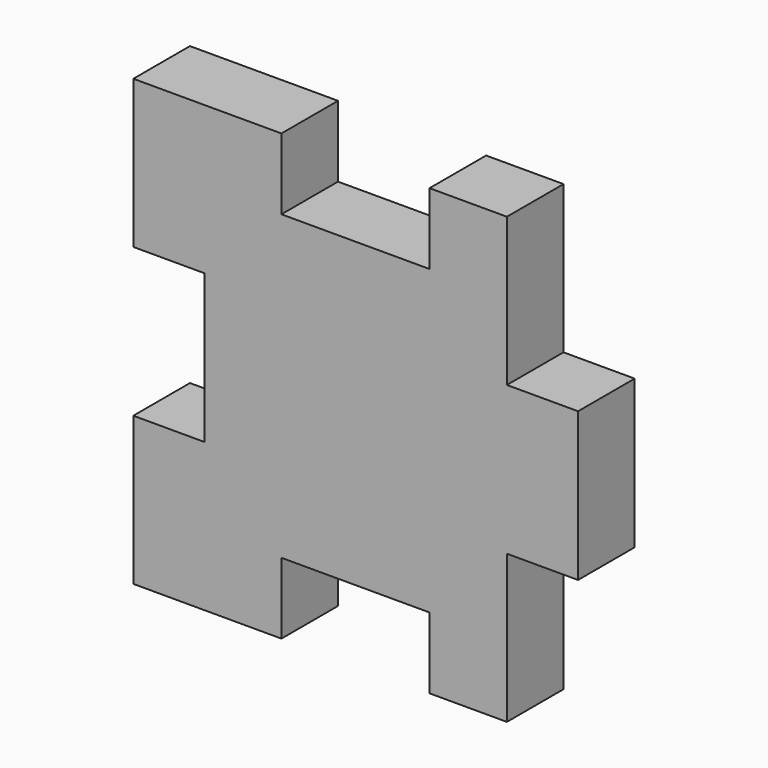
from build123d import *

# Parameters (mm, degrees)
F1_DEPTH     = 2.032
F3_TEXT_SIZE = 8.3215777159
F4_DEPTH     = 0.508


# Not quite as in the source:
# - Text() gives the source's letters only with a copy of the font that has no kerning and outlines rounded to 1/6400 em; it was checked with that copy


with BuildPart() as f1:
    # F0 (on Front) → F1 (new body)
    with BuildSketch(Plane.XZ):
        Polygon((-10.9897290399, 29.0234165891), (-10.9897290399, 26.8898165891), (-10.9897290399, 24.7562165891), (-13.0344290399, 24.7562165891), (-13.0344290399, 20.5017165891), (-8.7799290399, 20.5017165891), (-8.7799290399, 22.5464165891), (-4.5254290399, 22.5464165891), (-4.5254290399, 20.5017165891), (-2.3029290399, 20.5017165891), (-2.3029290399, 24.7562165891), (-0.2582290399, 24.7562165891), (-0.2582290399, 29.0234165891), (-2.3029290399, 29.0234165891), (-2.3029290399, 33.2779165891), (-4.5254290399, 33.2779165891), (-4.5254290399, 31.2332165891), (-8.7799290399, 31.2332165891), (-8.7799290399, 33.2779165891), (-13.0344290399, 33.2779165891), (-13.0344290399, 29.0234165891), align=None)
    extrude(amount=F1_DEPTH)

    # F3 (on offset) → F4 (cut)
    with BuildSketch(Plane.XZ.offset(4.064)):
        with Locations((-9.0134641383, 24.110636179)):
            Text('L', F3_TEXT_SIZE, font='Open Sans', text_align=(TextAlign.LEFT, TextAlign.BOTTOM))
    extrude(amount=-F4_DEPTH, mode=Mode.SUBTRACT)


solid = f1.part
